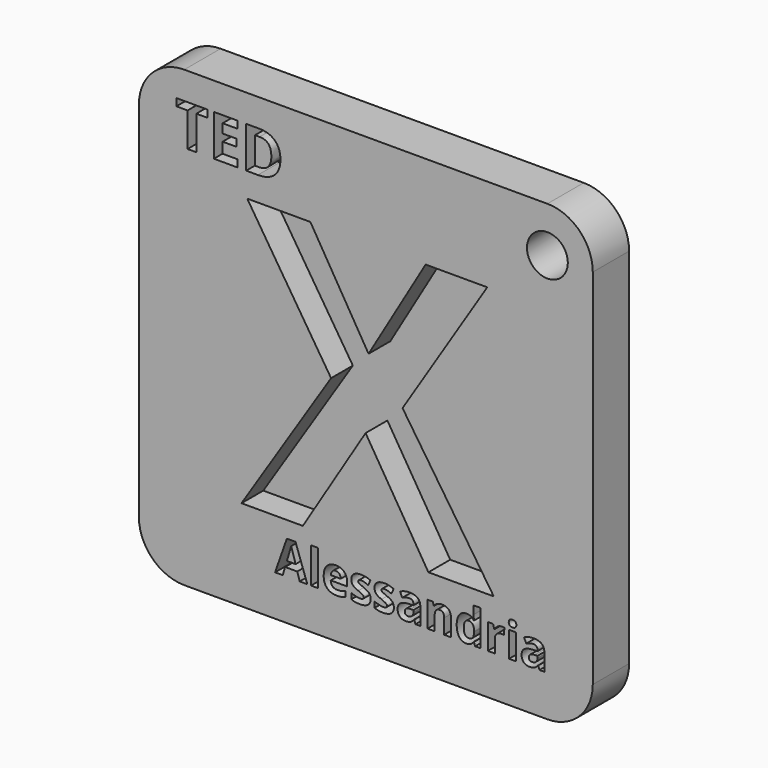
from build123d import *

# Parameters (mm, degrees)
F0_W         = 1270
F0_H         = 1270
F1_DEPTH     = 127
F2_TEXT_SIZE = 1058.3333333333
F3_DEPTH     = 76.2
F4_TEXT_SIZE = 130.7733562158
F5_DEPTH     = 76.2
F6_TEXT_SIZE = 161.6038439235
F7_DEPTH     = 76.2
F8_R         = 127
F9_R         = 57.15
F10_DEPTH    = 127


# Not quite as in the source:
# - Text() gives the source's letters only with a copy of the font that has no kerning and outlines rounded to 1/6400 em; it was checked with that copy


with BuildPart() as f1:
    # F0 (on Front) → F1 (new body)
    with BuildSketch(Plane.XZ):
        Rectangle(F0_W, F0_H)
    extrude(amount=F1_DEPTH)

    # F2 (on face) → F3 (cut)
    with BuildSketch(Plane.XZ.offset(127)):
        with Locations((-347.98, -381)):
            Text('X', F2_TEXT_SIZE, font='Open Sans', font_style=FontStyle.BOLD, text_align=(TextAlign.LEFT, TextAlign.BOTTOM))
    extrude(amount=-F3_DEPTH, mode=Mode.SUBTRACT)

    # F4 (on face) → F5 (cut)
    with BuildSketch(Plane.XZ.offset(127)):
        with Locations((-254, -520.7)):
            Text('Alessandria', F4_TEXT_SIZE, font='Open Sans', font_style=FontStyle.BOLD, text_align=(TextAlign.LEFT, TextAlign.BOTTOM))
    extrude(amount=-F5_DEPTH, mode=Mode.SUBTRACT)

    # F6 (on face) → F7 (cut)
    with BuildSketch(Plane.XZ.offset(127)):
        with Locations((-533.4, 442.4452323751)):
            Text('TED', F6_TEXT_SIZE, font='Open Sans', font_style=FontStyle.BOLD, text_align=(TextAlign.LEFT, TextAlign.BOTTOM))
    extrude(amount=-F7_DEPTH, mode=Mode.SUBTRACT)

    # F8
    f8_edges = [f1.edges().sort_by_distance(p)[0] for p in [
        (635, -63.5, 635),
        (-635, -63.5, 635),
        (-635, -63.5, -635),
        (635, -63.5, -635),
    ]]
    fillet(f8_edges, radius=F8_R)

    # F9 (on face) → F10 (cut, through all)
    with BuildSketch(Plane.XZ.offset(127)):
        with Locations((508, 508)):
            Circle(F9_R)
    extrude(amount=-F10_DEPTH, mode=Mode.SUBTRACT)


solid = f1.part
